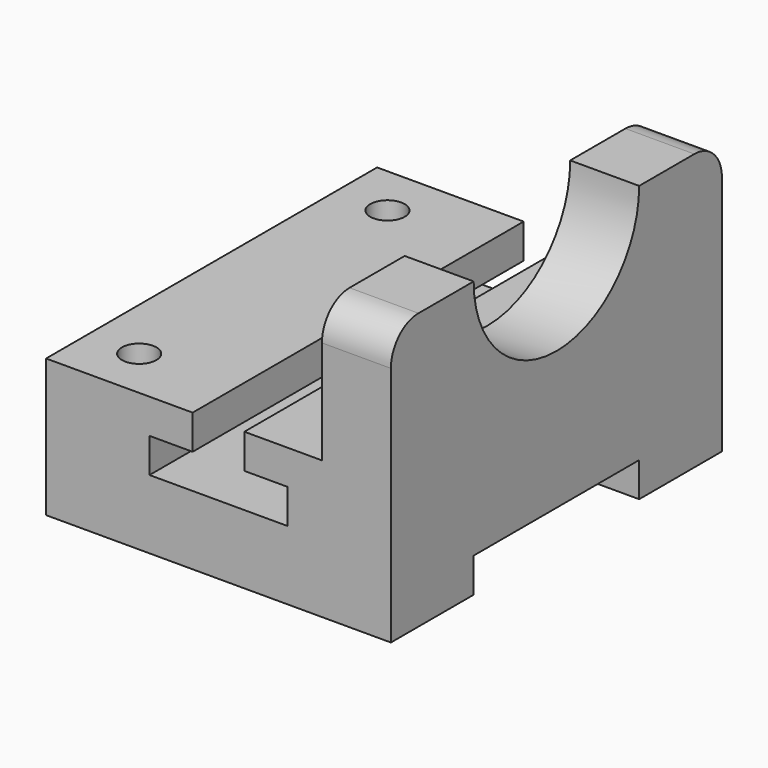
from build123d import *

# Parameters (mm, degrees)
F0_W      = 5
F0_H      = 4
F1_DEPTH  = 6
F2_W      = 4
F2_H      = 2
F3_DEPTH  = 6.001
F4_W      = 0.75
F4_H      = 0.5
F5_DEPTH  = 6.001
F6_W      = 3
F6_H      = 0.5
F7_DEPTH  = 5.001
F8_R      = 1.5
F9_DEPTH  = 1.001
F10_R     = 0.5
F11_R     = 0.25
F12_DEPTH = 2.001


# Not quite as in the source:
# - a pattern or mirror of a feature is missing from the dataset's text; its kind, count and spacing are read off the source's solid


with BuildPart() as f1:
    # F0 (on Front) → F1 (new body)
    with BuildSketch(Plane.XZ):
        Rectangle(F0_W, F0_H)
    extrude(amount=F1_DEPTH)

    # F2 (on face) → F3 (cut, through all)
    with BuildSketch(Plane.XZ.offset(6)):
        with Locations((-0.5, 1)):
            Rectangle(F2_W, F2_H)
    extrude(amount=-F3_DEPTH, mode=Mode.SUBTRACT)

    # F4 (on face) → F5 (cut, through all)
    with BuildSketch(Plane.XZ.offset(6)):
        with Locations((0, -0.25)):
            Rectangle(F4_W, F4_H)
        Polygon((1, -0.5), (0.375, -0.5), (-0.375, -0.5), (-1, -0.5), (-1, -1), (1, -1), align=None)
    extrude(amount=-F5_DEPTH, mode=Mode.SUBTRACT)

    # F6 (on face) → F7 (cut, through all)
    with BuildSketch(Plane(origin=(-2.5, 0, 0), x_dir=(0, -1, 0), z_dir=(-1, 0, 0))):
        with Locations((3, -1.75)):
            Rectangle(F6_W, F6_H)
    extrude(amount=-F7_DEPTH, mode=Mode.SUBTRACT)

    # F8 (on face) → F9 (cut, through all)
    with BuildSketch(Plane(origin=(1.5, 0, 0), x_dir=(0, -1, 0), z_dir=(-1, 0, 0))):
        with Locations((3, 2)):
            Circle(F8_R)
    extrude(amount=-F9_DEPTH, mode=Mode.SUBTRACT)

    # F10
    f10_edges = [f1.edges().sort_by_distance(p)[0] for p in [
        (2, -6, 2),
        (2, 0, 2),
    ]]
    fillet(f10_edges, radius=F10_R)

    # F11 (on face) → F12 (cut, through all)
    with BuildSketch(Plane.XY):
        with Locations((-1.75, -0.75)):
            Circle(F11_R)
    f12 = extrude(amount=-F12_DEPTH, mode=Mode.SUBTRACT)

    # F12_copies: F12 across plane
    add(f12.mirror(Plane(origin=(0, -3, 0), x_dir=(0, 0, -1), z_dir=(0, -1, 0))), mode=Mode.SUBTRACT)


solid = f1.part
